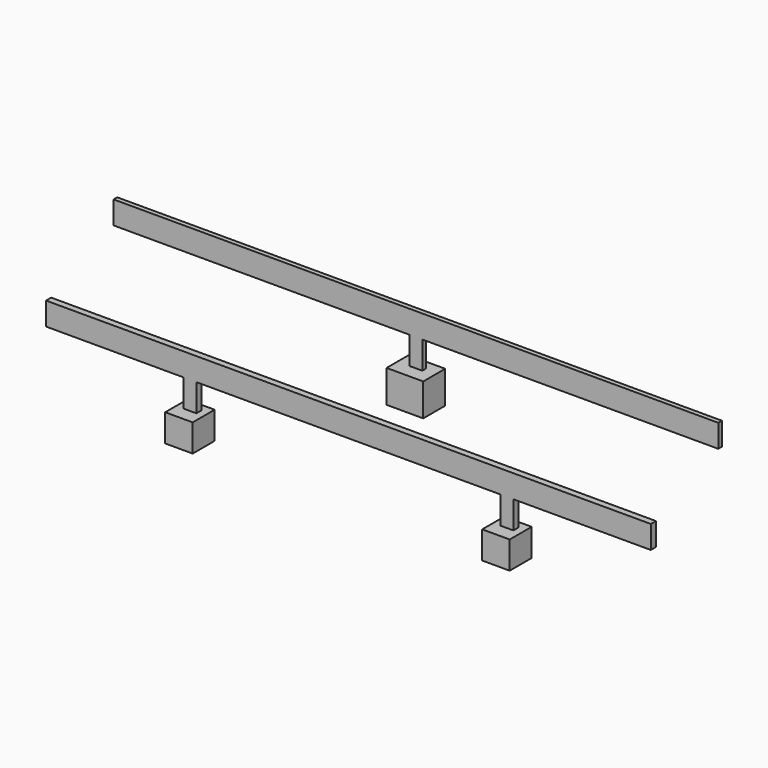
from build123d import *

# Parameters (mm, degrees)
F0_W     = 14
F0_H     = 30
F1_DEPTH = 7
F2_DEPTH = 15
F3_W     = 14
F3_H     = 30
F4_DEPTH = 5
F5_DEPTH = 15


with BuildPart() as f1:
    # F0 (on Front) → F1 (new body)
    with BuildSketch(Plane.XZ):
        Polygon((330, 200.8922785521), (-330, 200.8922785521), (-330, 175.8922785521), (-180, 175.8922785521), (-166, 175.8922785521), (166, 175.8922785521), (180, 175.8922785521), (330, 175.8922785521), align=None)
        with Locations((-173, 160.8922785521)):
            Rectangle(F0_W, F0_H)
        with Locations((173, 160.8922785521)):
            Rectangle(F0_W, F0_H)
    extrude(amount=-F1_DEPTH)

    # F0 (on Front) → F2 (join, symmetric)
    with BuildSketch(Plane.XZ):
        Polygon((-166, 145.8922785521), (-180, 145.8922785521), (-188, 145.8922785521), (-188, 115.8922785521), (-158, 115.8922785521), (-158, 145.8922785521), align=None)
        Polygon((188, 145.8922785521), (180, 145.8922785521), (166, 145.8922785521), (158, 145.8922785521), (158, 115.8922785521), (188, 115.8922785521), align=None)
    extrude(amount=F2_DEPTH, both=True)


with BuildPart() as f4:
    # F3 (on Front) → F4 (new body)
    with BuildSketch(Plane.XZ):
        Polygon((172.8154140711, 261.3809283972), (-487.1845859289, 261.3809283972), (-487.1845859289, 236.3809283972), (-164.1845859289, 236.3809283972), (-150.1845859289, 236.3809283972), (172.8154140711, 236.3809283972), align=None)
        with Locations((-157.1845859289, 221.3809283972)):
            Rectangle(F3_W, F3_H)
    extrude(amount=-F4_DEPTH)

    # F3 (on Front) → F5 (join, symmetric)
    with BuildSketch(Plane.XZ):
        Polygon((-150.1845859289, 206.3809283972), (-164.1845859289, 206.3809283972), (-177.1845859289, 206.3809283972), (-177.1845859289, 170.889923811), (-137.1845859289, 170.889923811), (-137.1845859289, 206.3809283972), align=None)
    extrude(amount=F5_DEPTH, both=True)


with BuildPart() as f4_1:
    # F6: moved
    add(f4.part.moved(Location((158, 91, 0))))


solid = Compound([f1.part, f4_1.part])
